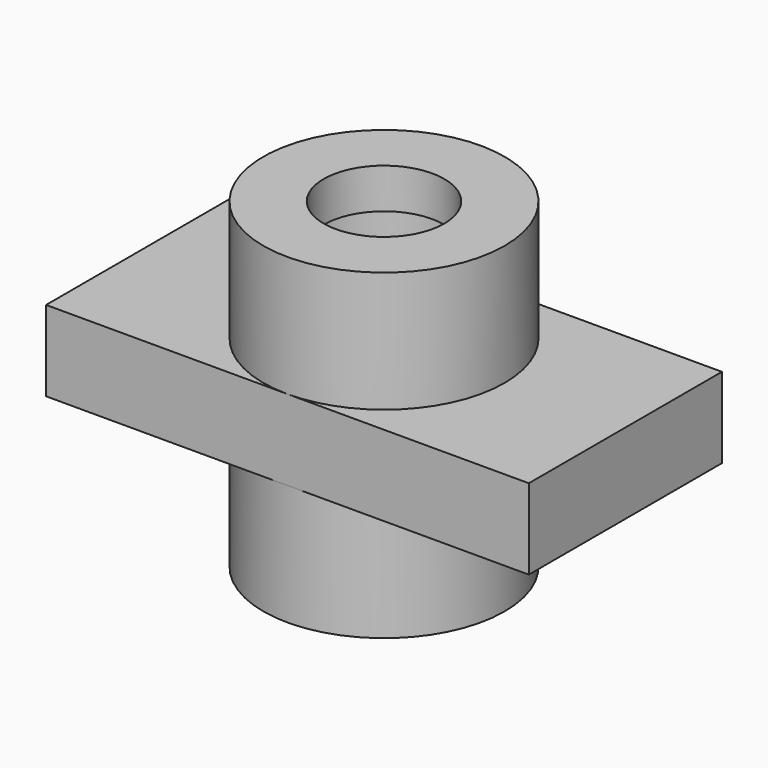
from build123d import *

# Parameters (mm, degrees)
F0_W     = 9.525
F0_H     = 6.35
F0_H_2   = 12.7
F0_H_3   = 19.05
F3_DEPTH = 31.751
F5_DEPTH = 12.7
F6_W     = 9.525
F6_H     = 6.35
F6_H_2   = 38.1


# Not quite as in the source:
# - an extrude ends at something that could not be found from the text; its depth is read off the source's solid


with BuildPart() as f1:
    # F0 (on Front) → F1 (revolve)
    with BuildSketch(Plane.XZ):
        with Locations((4.7625, 47.625)):
            Rectangle(F0_W, F0_H)
        Polygon((19.05, 50.8), (9.525, 50.8), (9.525, 44.45), (12.7, 44.45), (12.7, 38.1), (9.525, 38.1), (9.525, 31.75), (19.05, 31.75), align=None)
        Polygon((9.525, 44.45), (0, 44.45), (0, 38.1), (9.525, 38.1), (12.7, 38.1), (12.7, 44.45), align=None)
        with Locations((4.7625, 34.925)):
            Rectangle(F0_W, F0_H)
        Polygon((38.1, 31.75), (19.05, 31.75), (9.525, 31.75), (9.525, 19.05), (19.05, 19.05), (38.1, 19.05), align=None)
        with Locations((4.7625, 25.4)):
            Rectangle(F0_W, F0_H_2)
        with Locations((4.7625, 9.525)):
            Rectangle(F0_W, F0_H_3)
        with Locations((14.2875, 9.525)):
            Rectangle(F0_W, F0_H_3)
    revolve(axis=Axis((0, 0, 25.4), (0, 0, 1)))

    # F2 (on face) → F3 (cut, through all)
    with BuildSketch(Plane.XY.offset(31.75)):
        with BuildLine():
            ThreePointArc((32.9955678842, 19.05), (0, 38.1), (-32.9955678842, 19.05))
            Line((-32.9955678842, 19.05), (3.68e-08, 19.05))
            Line((3.68e-08, 19.05), (32.9955678842, 19.05))
        make_face()
        with BuildLine():
            Line((3.68e-08, -19.05), (-32.9955678842, -19.05))
            ThreePointArc((-32.9955678842, -19.05), (0, -38.1), (32.9955678842, -19.05))
            Line((32.9955678842, -19.05), (3.68e-08, -19.05))
        make_face()
    extrude(amount=-F3_DEPTH, mode=Mode.SUBTRACT)

    # F4 (on face) → F5 (join, through all)
    with BuildSketch(Plane.XY.offset(31.75)):
        with BuildLine():
            ThreePointArc((-38.1, 0), (-36.8017739816, 9.8610056184), (-32.9955678842, 19.05))
            Line((-32.9955678842, 19.05), (-38.1, 19.05))
            Line((-38.1, 19.05), (-38.1, 0))
        make_face()
        with BuildLine():
            ThreePointArc((-32.9955678842, -19.05), (-36.8017739816, -9.8610056184), (-38.1, 0))
            Line((-38.1, 0), (-38.1, -19.05))
            Line((-38.1, -19.05), (-32.9955678842, -19.05))
        make_face()
        with BuildLine():
            Line((38.1, 0), (38.1, 19.05))
            Line((38.1, 19.05), (32.9955678842, 19.05))
            ThreePointArc((32.9955678842, 19.05), (36.8017739816, 9.8610056184), (38.1, 0))
        make_face()
        with BuildLine():
            Line((38.1, -19.05), (38.1, 0))
            ThreePointArc((38.1, 0), (36.8017739816, -9.8610056184), (32.9955678842, -19.05))
            Line((32.9955678842, -19.05), (38.1, -19.05))
        make_face()
    extrude(amount=-F5_DEPTH)

    # F6 (on Front) → F7 (revolve, cut)
    with BuildSketch(Plane.XZ):
        with Locations((4.7625, 47.625)):
            Rectangle(F6_W, F6_H)
        Polygon((9.525, 44.45), (0, 44.45), (0, 38.1), (9.525, 38.1), (12.7, 38.1), (12.7, 44.45), align=None)
        with Locations((4.7625, 19.05)):
            Rectangle(F6_W, F6_H_2)
    revolve(axis=Axis((0, 0, 30.4315376466), (0, 0, 1)), mode=Mode.SUBTRACT)


solid = f1.part
